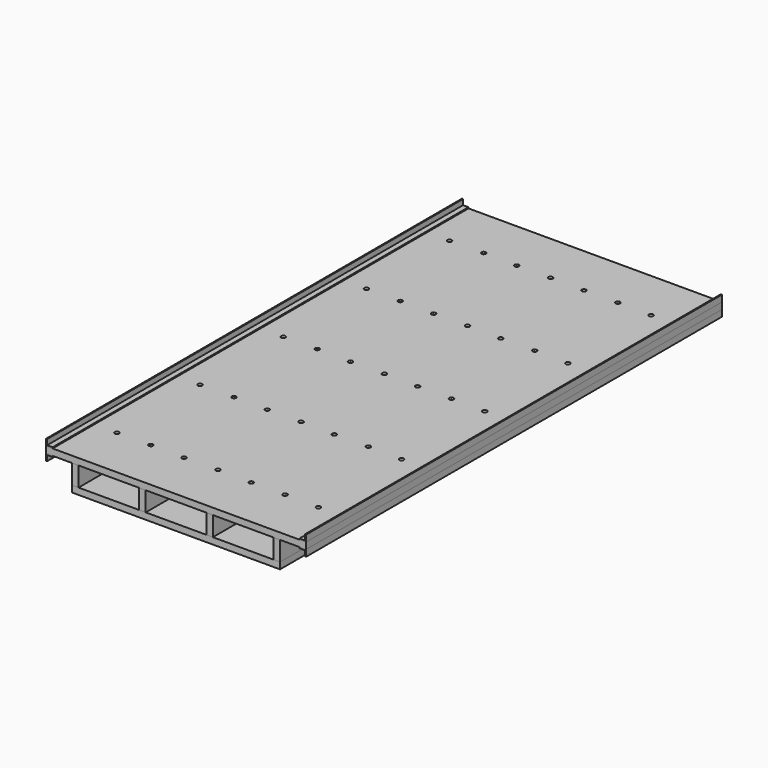
from build123d import *

# Parameters (mm, degrees)
F0_W                     = 762
F0_H                     = 1524
F1_DEPTH                 = 19.05
F3_START                 = -19.05
F2_W                     = 19.05
F2_H                     = 1524
F3_DEPTH                 = 57.15
F5_START                 = -19.05
F4_W                     = 571.5
F4_H                     = 19.05
F5_DEPTH                 = 57.15
F6_W                     = 19.05
F6_H                     = 28.575
F7_DEPTH                 = 1379.856
F11_D                    = 4.7625
F11_DEPTH                = 38.1
F11_CSINK_D              = 12.7
F11_CSINK_ANGLE          = 90
F11_TIP                  = 1.4307993491
F11_2_D                  = 4.7625
F11_2_DEPTH              = 38.1
F11_2_CSINK_D            = 12.7
F11_2_CSINK_ANGLE        = 90
F11_2_TIP                = 1.4307993491
F11_3_D                  = 4.7625
F11_3_DEPTH              = 38.1
F11_3_CSINK_D            = 12.7
F11_3_CSINK_ANGLE        = 90
F11_3_TIP                = 1.4307993491
F11_4_D                  = 4.7625
F11_4_DEPTH              = 38.1
F11_4_CSINK_D            = 12.7
F11_4_CSINK_ANGLE        = 90
F11_4_TIP                = 1.4307993491
F11_5_D                  = 4.7625
F11_5_DEPTH              = 38.1
F11_5_CSINK_D            = 12.7
F11_5_CSINK_ANGLE        = 90
F11_5_TIP                = 1.4307993491
F11_ON_F10_D             = 4.7625
F11_ON_F10_DEPTH         = 38.1
F11_ON_F10_CSINK_D       = 12.7
F11_ON_F10_CSINK_ANGLE   = 90
F11_ON_F10_TIP           = 1.4307993491
F12_W                    = 609.6
F12_H                    = 1524
F13_DEPTH                = 19.05
F15_D                    = 4.7625
F15_DEPTH                = 38.1
F15_CSINK_D              = 12.7
F15_CSINK_ANGLE          = 90
F15_TIP                  = 1.4307993491
F15_2_D                  = 4.7625
F15_2_DEPTH              = 38.1
F15_2_CSINK_D            = 12.7
F15_2_CSINK_ANGLE        = 90
F15_2_TIP                = 1.4307993491
F15_3_D                  = 4.7625
F15_3_DEPTH              = 38.1
F15_3_CSINK_D            = 12.7
F15_3_CSINK_ANGLE        = 90
F15_3_TIP                = 1.4307993491
F15_4_D                  = 4.7625
F15_4_DEPTH              = 38.1
F15_4_CSINK_D            = 12.7
F15_4_CSINK_ANGLE        = 90
F15_4_TIP                = 1.4307993491
F15_5_D                  = 4.7625
F15_5_DEPTH              = 38.1
F15_5_CSINK_D            = 12.7
F15_5_CSINK_ANGLE        = 90
F15_5_TIP                = 1.4307993491
F15_6_D                  = 4.7625
F15_6_DEPTH              = 38.1
F15_6_CSINK_D            = 12.7
F15_6_CSINK_ANGLE        = 90
F15_6_TIP                = 1.4307993491
F15_7_D                  = 4.7625
F15_7_DEPTH              = 38.1
F15_7_CSINK_D            = 12.7
F15_7_CSINK_ANGLE        = 90
F15_7_TIP                = 1.4307993491
F15_8_D                  = 4.7625
F15_8_DEPTH              = 38.1
F15_8_CSINK_D            = 12.7
F15_8_CSINK_ANGLE        = 90
F15_8_TIP                = 1.4307993491
F17_D                    = 4.7625
F17_DEPTH                = 38.1
F17_CSINK_D              = 12.7
F17_CSINK_ANGLE          = 90
F17_TIP                  = 1.4307993491
F17_2_D                  = 4.7625
F17_2_DEPTH              = 38.1
F17_2_CSINK_D            = 12.7
F17_2_CSINK_ANGLE        = 90
F17_2_TIP                = 1.4307993491
F17_3_D                  = 4.7625
F17_3_DEPTH              = 38.1
F17_3_CSINK_D            = 12.7
F17_3_CSINK_ANGLE        = 90
F17_3_TIP                = 1.4307993491
F17_4_D                  = 4.7625
F17_4_DEPTH              = 38.1
F17_4_CSINK_D            = 12.7
F17_4_CSINK_ANGLE        = 90
F17_4_TIP                = 1.4307993491
F17_5_D                  = 4.7625
F17_5_DEPTH              = 38.1
F17_5_CSINK_D            = 12.7
F17_5_CSINK_ANGLE        = 90
F17_5_TIP                = 1.4307993491
F17_6_D                  = 4.7625
F17_6_DEPTH              = 38.1
F17_6_CSINK_D            = 12.7
F17_6_CSINK_ANGLE        = 90
F17_6_TIP                = 1.4307993491
F19_D                    = 4.7625
F19_DEPTH                = 38.1
F19_START                = 19.05
F19_CSINK_D              = 12.7
F19_CSINK_ANGLE          = 90
F19_TIP                  = 1.4307993491
F19_2_D                  = 4.7625
F19_2_DEPTH              = 38.1
F19_2_START              = 19.05
F19_2_CSINK_D            = 12.7
F19_2_CSINK_ANGLE        = 90
F19_2_TIP                = 1.4307993491
F19_3_D                  = 4.7625
F19_3_DEPTH              = 38.1
F19_3_START              = 19.05
F19_3_CSINK_D            = 12.7
F19_3_CSINK_ANGLE        = 90
F19_3_TIP                = 1.4307993491
F19_4_D                  = 4.7625
F19_4_DEPTH              = 38.1
F19_4_START              = 19.05
F19_4_CSINK_D            = 12.7
F19_4_CSINK_ANGLE        = 90
F19_4_TIP                = 1.4307993491
F19_5_D                  = 4.7625
F19_5_DEPTH              = 38.1
F19_5_START              = 19.05
F19_5_CSINK_D            = 12.7
F19_5_CSINK_ANGLE        = 90
F19_5_TIP                = 1.4307993491
F19_ON_F18_D             = 4.7625
F19_ON_F18_DEPTH         = 38.1
F19_ON_F18_CSINK_D       = 12.7
F19_ON_F18_CSINK_ANGLE   = 90
F19_ON_F18_TIP           = 1.4307993491
F19_ON_F18_2_D           = 4.7625
F19_ON_F18_2_DEPTH       = 38.1
F19_ON_F18_2_CSINK_D     = 12.7
F19_ON_F18_2_CSINK_ANGLE = 90
F19_ON_F18_2_TIP         = 1.4307993491
F19_ON_F18_3_D           = 4.7625
F19_ON_F18_3_DEPTH       = 38.1
F19_ON_F18_3_CSINK_D     = 12.7
F19_ON_F18_3_CSINK_ANGLE = 90
F19_ON_F18_3_TIP         = 1.4307993491
F19_ON_F18_4_D           = 4.7625
F19_ON_F18_4_DEPTH       = 38.1
F19_ON_F18_4_CSINK_D     = 12.7
F19_ON_F18_4_CSINK_ANGLE = 90
F19_ON_F18_4_TIP         = 1.4307993491
F19_ON_F18_5_D           = 4.7625
F19_ON_F18_5_DEPTH       = 38.1
F19_ON_F18_5_CSINK_D     = 12.7
F19_ON_F18_5_CSINK_ANGLE = 90
F19_ON_F18_5_TIP         = 1.4307993491
F19_ON_F18_6_D           = 4.7625
F19_ON_F18_6_DEPTH       = 38.1
F19_ON_F18_6_CSINK_D     = 12.7
F19_ON_F18_6_CSINK_ANGLE = 90
F19_ON_F18_6_TIP         = 1.4307993491
F21_DEPTH                = 1524


# Not quite as in the source:
# - a feature names something its author has since deleted; it is built from what else it names


with BuildPart() as f1:
    # F0 (on Top) → F1 (new body)
    with BuildSketch(Plane.XY):
        with Locations((381, 762)):
            Rectangle(F0_W, F0_H)
    extrude(amount=-F1_DEPTH)

    # F11
    with Locations(Plane.XY):
        with Locations((85.725, 457.2), (85.725, 762), (85.725, 1066.8), (85.725, 1371.6), (676.275, 1066.8), (479.425, 1371.6), (479.425, 1066.8), (479.425, 762), (479.425, 457.2), (282.575, 1371.6), (479.425, 152.4), (676.275, 457.2), (282.575, 762), (676.275, 152.4), (282.575, 1066.8), (282.575, 152.4), (676.275, 762), (282.575, 457.2), (676.275, 1371.6), (85.725, 152.4)):
            CounterSinkHole(F11_D / 2, F11_CSINK_D / 2, depth=F11_DEPTH, counter_sink_angle=F11_CSINK_ANGLE)
            with Locations((0, 0, -(F11_DEPTH + F11_TIP / 2))):  # 118° drill point
                Cone(0, F11_D / 2, F11_TIP, mode=Mode.SUBTRACT)

    # F11 on F10
    with Locations(Plane.XY):
        with Locations((184.15, 1068.07), (381, 1372.87), (381, 153.67), (577.85, 1372.87), (381, 763.27), (184.15, 458.47), (184.15, 763.27), (577.85, 153.67), (577.85, 763.27), (381, 458.47), (184.15, 153.67), (577.85, 458.47), (184.15, 1372.87), (577.85, 1068.07), (381, 1068.07)):
            CounterSinkHole(F11_ON_F10_D / 2, F11_ON_F10_CSINK_D / 2, depth=F11_ON_F10_DEPTH, counter_sink_angle=F11_ON_F10_CSINK_ANGLE)
            with Locations((0, 0, -(F11_ON_F10_DEPTH + F11_ON_F10_TIP / 2))):  # 118° drill point
                Cone(0, F11_ON_F10_D / 2, F11_ON_F10_TIP, mode=Mode.SUBTRACT)


with BuildPart() as f3:
    # F2 (on face) → F3 (new body)
    with BuildSketch(Plane.XY.offset(F3_START)):
        with Locations((85.725, 762)):
            Rectangle(F2_W, F2_H)
    extrude(amount=-F3_DEPTH)

    # F11#2
    with Locations(Plane.XY):
        with Locations((85.725, 457.2), (85.725, 762), (85.725, 1066.8), (85.725, 1371.6), (676.275, 1066.8), (479.425, 1371.6), (479.425, 1066.8), (479.425, 762), (479.425, 457.2), (282.575, 1371.6), (479.425, 152.4), (676.275, 457.2), (282.575, 762), (676.275, 152.4), (282.575, 1066.8), (282.575, 152.4), (676.275, 762), (282.575, 457.2), (676.275, 1371.6), (85.725, 152.4)):
            CounterSinkHole(F11_2_D / 2, F11_2_CSINK_D / 2, depth=F11_2_DEPTH, counter_sink_angle=F11_2_CSINK_ANGLE)
            with Locations((0, 0, -(F11_2_DEPTH + F11_2_TIP / 2))):  # 118° drill point
                Cone(0, F11_2_D / 2, F11_2_TIP, mode=Mode.SUBTRACT)

    # F15
    with Locations(Plane(origin=(0, 0, -95.25), x_dir=(1, 0, 0), z_dir=(0, 0, -1))):
        with Locations((184.15, -152.4), (381, -458.47), (381, -763.27), (676.275, -762), (184.15, -458.47), (282.575, -762), (381, -153.67), (479.425, -762), (282.575, -457.2), (676.275, -457.2), (479.425, -457.2), (577.85, -153.67), (479.425, -152.4), (676.275, -152.4), (282.575, -153.67), (577.85, -458.47), (577.85, -763.27), (282.575, -1371.6), (676.275, -1066.8), (85.725, -1066.8), (479.425, -1371.6), (85.725, -152.4), (479.425, -1066.8), (577.85, -1372.87), (282.575, -1066.8), (381, -1068.07), (381, -1372.87), (85.725, -762), (577.85, -1068.07), (85.725, -457.2), (184.15, -1372.87), (85.725, -1371.6), (676.275, -1371.6), (184.15, -1068.07), (184.15, -762)):
            CounterSinkHole(F15_D / 2, F15_CSINK_D / 2, depth=F15_DEPTH, counter_sink_angle=F15_CSINK_ANGLE)
            with Locations((0, 0, -(F15_DEPTH + F15_TIP / 2))):  # 118° drill point
                Cone(0, F15_D / 2, F15_TIP, mode=Mode.SUBTRACT)

    # F17
    with Locations(Plane(origin=(76.2, 0, 0), x_dir=(0, -1, 0), z_dir=(-1, 0, 0))):
        with Locations((-458.47, -57.15), (-1372.87, -38.1), (-1372.87, -57.15), (-458.47, -38.1), (-1068.07, -57.15), (-763.27, -38.1), (-153.67, -57.15), (-1068.07, -38.1), (-763.27, -57.15), (-153.67, -38.1)):
            CounterSinkHole(F17_D / 2, F17_CSINK_D / 2, depth=F17_DEPTH, counter_sink_angle=F17_CSINK_ANGLE)
            with Locations((0, 0, -(F17_DEPTH + F17_TIP / 2))):  # 118° drill point
                Cone(0, F17_D / 2, F17_TIP, mode=Mode.SUBTRACT)


with BuildPart() as f3b:
    # F2 (on face) → F3, piece 2 (new body)
    with BuildSketch(Plane.XY.offset(F3_START)):
        with Locations((282.575, 762)):
            Rectangle(F2_W, F2_H)
    extrude(amount=-F3_DEPTH)


with BuildPart() as f3c:
    # F2 (on face) → F3, piece 3 (new body)
    with BuildSketch(Plane.XY.offset(F3_START)):
        with Locations((479.425, 762)):
            Rectangle(F2_W, F2_H)
    extrude(amount=-F3_DEPTH)


with BuildPart() as f3d:
    # F2 (on face) → F3, piece 4 (new body)
    with BuildSketch(Plane.XY.offset(F3_START)):
        with Locations((676.275, 762)):
            Rectangle(F2_W, F2_H)
    extrude(amount=-F3_DEPTH)

    # F11#5
    with Locations(Plane.XY):
        with Locations((85.725, 457.2), (85.725, 762), (85.725, 1066.8), (85.725, 1371.6), (676.275, 1066.8), (479.425, 1371.6), (479.425, 1066.8), (479.425, 762), (479.425, 457.2), (282.575, 1371.6), (479.425, 152.4), (676.275, 457.2), (282.575, 762), (676.275, 152.4), (282.575, 1066.8), (282.575, 152.4), (676.275, 762), (282.575, 457.2), (676.275, 1371.6), (85.725, 152.4)):
            CounterSinkHole(F11_5_D / 2, F11_5_CSINK_D / 2, depth=F11_5_DEPTH, counter_sink_angle=F11_5_CSINK_ANGLE)
            with Locations((0, 0, -(F11_5_DEPTH + F11_5_TIP / 2))):  # 118° drill point
                Cone(0, F11_5_D / 2, F11_5_TIP, mode=Mode.SUBTRACT)

    # F15#2
    with Locations(Plane(origin=(0, 0, -95.25), x_dir=(1, 0, 0), z_dir=(0, 0, -1))):
        with Locations((184.15, -152.4), (381, -458.47), (381, -763.27), (676.275, -762), (184.15, -458.47), (282.575, -762), (381, -153.67), (479.425, -762), (282.575, -457.2), (676.275, -457.2), (479.425, -457.2), (577.85, -153.67), (479.425, -152.4), (676.275, -152.4), (282.575, -153.67), (577.85, -458.47), (577.85, -763.27), (282.575, -1371.6), (676.275, -1066.8), (85.725, -1066.8), (479.425, -1371.6), (85.725, -152.4), (479.425, -1066.8), (577.85, -1372.87), (282.575, -1066.8), (381, -1068.07), (381, -1372.87), (85.725, -762), (577.85, -1068.07), (85.725, -457.2), (184.15, -1372.87), (85.725, -1371.6), (676.275, -1371.6), (184.15, -1068.07), (184.15, -762)):
            CounterSinkHole(F15_2_D / 2, F15_2_CSINK_D / 2, depth=F15_2_DEPTH, counter_sink_angle=F15_2_CSINK_ANGLE)
            with Locations((0, 0, -(F15_2_DEPTH + F15_2_TIP / 2))):  # 118° drill point
                Cone(0, F15_2_D / 2, F15_2_TIP, mode=Mode.SUBTRACT)

    # F19 on F18
    with Locations(Plane.YZ.offset(685.8)):
        with Locations((763.27, -38.1), (458.47, -38.1), (153.67, -57.15), (1068.07, -57.15), (153.67, -38.1), (458.47, -57.15), (1372.87, -38.1), (1372.87, -57.15), (1068.07, -38.1), (763.27, -57.15)):
            CounterSinkHole(F19_ON_F18_D / 2, F19_ON_F18_CSINK_D / 2, depth=F19_ON_F18_DEPTH, counter_sink_angle=F19_ON_F18_CSINK_ANGLE)
            with Locations((0, 0, -(F19_ON_F18_DEPTH + F19_ON_F18_TIP / 2))):  # 118° drill point
                Cone(0, F19_ON_F18_D / 2, F19_ON_F18_TIP, mode=Mode.SUBTRACT)


with BuildPart() as f5:
    # F4 (on face) → F5 (new body)
    with BuildSketch(Plane.XY.offset(F5_START)):
        with Locations((381, 153.67)):
            Rectangle(F4_W, F4_H)
    extrude(amount=-F5_DEPTH)


with BuildPart() as f5b:
    # F4 (on face) → F5, piece 2 (new body)
    with BuildSketch(Plane.XY.offset(F5_START)):
        with Locations((381, 763.27)):
            Rectangle(F4_W, F4_H)
    extrude(amount=-F5_DEPTH)


with BuildPart() as f5c:
    # F4 (on face) → F5, piece 3 (new body)
    with BuildSketch(Plane.XY.offset(F5_START)):
        with Locations((381, 1068.07)):
            Rectangle(F4_W, F4_H)
    extrude(amount=-F5_DEPTH)


with BuildPart() as f5d:
    # F4 (on face) → F5, piece 4 (new body)
    with BuildSketch(Plane.XY.offset(F5_START)):
        with Locations((381, 1372.87)):
            Rectangle(F4_W, F4_H)
    extrude(amount=-F5_DEPTH)


with BuildPart() as f5e:
    # F4 (on face) → F5, piece 5 (new body)
    with BuildSketch(Plane.XY.offset(F5_START)):
        with Locations((381, 458.47)):
            Rectangle(F4_W, F4_H)
    extrude(amount=-F5_DEPTH)


with BuildPart() as f7_tool:
    # F6 (on face) → F7 (new body, through all)
    with BuildSketch(Plane.XZ.offset(-144.145)):
        with Locations((282.575, -33.3375)):
            Rectangle(F6_W, F6_H)
        with Locations((479.425, -33.3375)):
            Rectangle(F6_W, F6_H)
    extrude(amount=-F7_DEPTH)


with BuildPart() as f5_1:
    add(f5.part)

    # F7: cut by f7_tool
    add(f7_tool.part, mode=Mode.SUBTRACT)


with BuildPart() as f5b_1:
    add(f5b.part)

    # F7: cut by f7_tool
    add(f7_tool.part, mode=Mode.SUBTRACT)


with BuildPart() as f5c_1:
    add(f5c.part)

    # F7: cut by f7_tool
    add(f7_tool.part, mode=Mode.SUBTRACT)


with BuildPart() as f5d_1:
    add(f5d.part)

    # F7: cut by f7_tool
    add(f7_tool.part, mode=Mode.SUBTRACT)


with BuildPart() as f5e_1:
    add(f5e.part)

    # F7: cut by f7_tool
    add(f7_tool.part, mode=Mode.SUBTRACT)


with BuildPart() as f3b_1:
    add(f3b.part)

    # F8: cut F5, F5e, F5b, F5c, F5d
    add(f5_1.part, mode=Mode.SUBTRACT)
    add(f5e_1.part, mode=Mode.SUBTRACT)
    add(f5b_1.part, mode=Mode.SUBTRACT)
    add(f5c_1.part, mode=Mode.SUBTRACT)
    add(f5d_1.part, mode=Mode.SUBTRACT)

    # F11#3
    with Locations(Plane.XY):
        with Locations((85.725, 457.2), (85.725, 762), (85.725, 1066.8), (85.725, 1371.6), (676.275, 1066.8), (479.425, 1371.6), (479.425, 1066.8), (479.425, 762), (479.425, 457.2), (282.575, 1371.6), (479.425, 152.4), (676.275, 457.2), (282.575, 762), (676.275, 152.4), (282.575, 1066.8), (282.575, 152.4), (676.275, 762), (282.575, 457.2), (676.275, 1371.6), (85.725, 152.4)):
            CounterSinkHole(F11_3_D / 2, F11_3_CSINK_D / 2, depth=F11_3_DEPTH, counter_sink_angle=F11_3_CSINK_ANGLE)
            with Locations((0, 0, -(F11_3_DEPTH + F11_3_TIP / 2))):  # 118° drill point
                Cone(0, F11_3_D / 2, F11_3_TIP, mode=Mode.SUBTRACT)


with BuildPart() as f3c_1:
    add(f3c.part)

    # F8: cut F5, F5e, F5b, F5c, F5d
    add(f5_1.part, mode=Mode.SUBTRACT)
    add(f5e_1.part, mode=Mode.SUBTRACT)
    add(f5b_1.part, mode=Mode.SUBTRACT)
    add(f5c_1.part, mode=Mode.SUBTRACT)
    add(f5d_1.part, mode=Mode.SUBTRACT)

    # F11#4
    with Locations(Plane.XY):
        with Locations((85.725, 457.2), (85.725, 762), (85.725, 1066.8), (85.725, 1371.6), (676.275, 1066.8), (479.425, 1371.6), (479.425, 1066.8), (479.425, 762), (479.425, 457.2), (282.575, 1371.6), (479.425, 152.4), (676.275, 457.2), (282.575, 762), (676.275, 152.4), (282.575, 1066.8), (282.575, 152.4), (676.275, 762), (282.575, 457.2), (676.275, 1371.6), (85.725, 152.4)):
            CounterSinkHole(F11_4_D / 2, F11_4_CSINK_D / 2, depth=F11_4_DEPTH, counter_sink_angle=F11_4_CSINK_ANGLE)
            with Locations((0, 0, -(F11_4_DEPTH + F11_4_TIP / 2))):  # 118° drill point
                Cone(0, F11_4_D / 2, F11_4_TIP, mode=Mode.SUBTRACT)


with BuildPart() as f13:
    # F12 (on face) → F13 (new body)
    with BuildSketch(Plane(origin=(0, 0, -76.2), x_dir=(1, 0, 0), z_dir=(0, 0, -1))):
        with Locations((381, -762)):
            Rectangle(F12_W, F12_H)
    extrude(amount=F13_DEPTH)

    # F15#8
    with Locations(Plane(origin=(0, 0, -95.25), x_dir=(1, 0, 0), z_dir=(0, 0, -1))):
        with Locations((184.15, -152.4), (381, -458.47), (381, -763.27), (676.275, -762), (184.15, -458.47), (282.575, -762), (381, -153.67), (479.425, -762), (282.575, -457.2), (676.275, -457.2), (479.425, -457.2), (577.85, -153.67), (479.425, -152.4), (676.275, -152.4), (282.575, -153.67), (577.85, -458.47), (577.85, -763.27), (282.575, -1371.6), (676.275, -1066.8), (85.725, -1066.8), (479.425, -1371.6), (85.725, -152.4), (479.425, -1066.8), (577.85, -1372.87), (282.575, -1066.8), (381, -1068.07), (381, -1372.87), (85.725, -762), (577.85, -1068.07), (85.725, -457.2), (184.15, -1372.87), (85.725, -1371.6), (676.275, -1371.6), (184.15, -1068.07), (184.15, -762)):
            CounterSinkHole(F15_8_D / 2, F15_8_CSINK_D / 2, depth=F15_8_DEPTH, counter_sink_angle=F15_8_CSINK_ANGLE)
            with Locations((0, 0, -(F15_8_DEPTH + F15_8_TIP / 2))):  # 118° drill point
                Cone(0, F15_8_D / 2, F15_8_TIP, mode=Mode.SUBTRACT)


with BuildPart() as f5_2:
    add(f5_1.part)

    # F15#3
    with Locations(Plane(origin=(0, 0, -95.25), x_dir=(1, 0, 0), z_dir=(0, 0, -1))):
        with Locations((184.15, -152.4), (381, -458.47), (381, -763.27), (676.275, -762), (184.15, -458.47), (282.575, -762), (381, -153.67), (479.425, -762), (282.575, -457.2), (676.275, -457.2), (479.425, -457.2), (577.85, -153.67), (479.425, -152.4), (676.275, -152.4), (282.575, -153.67), (577.85, -458.47), (577.85, -763.27), (282.575, -1371.6), (676.275, -1066.8), (85.725, -1066.8), (479.425, -1371.6), (85.725, -152.4), (479.425, -1066.8), (577.85, -1372.87), (282.575, -1066.8), (381, -1068.07), (381, -1372.87), (85.725, -762), (577.85, -1068.07), (85.725, -457.2), (184.15, -1372.87), (85.725, -1371.6), (676.275, -1371.6), (184.15, -1068.07), (184.15, -762)):
            CounterSinkHole(F15_3_D / 2, F15_3_CSINK_D / 2, depth=F15_3_DEPTH, counter_sink_angle=F15_3_CSINK_ANGLE)
            with Locations((0, 0, -(F15_3_DEPTH + F15_3_TIP / 2))):  # 118° drill point
                Cone(0, F15_3_D / 2, F15_3_TIP, mode=Mode.SUBTRACT)

    # F17#2
    with Locations(Plane(origin=(76.2, 0, 0), x_dir=(0, -1, 0), z_dir=(-1, 0, 0))):
        with Locations((-458.47, -57.15), (-1372.87, -38.1), (-1372.87, -57.15), (-458.47, -38.1), (-1068.07, -57.15), (-763.27, -38.1), (-153.67, -57.15), (-1068.07, -38.1), (-763.27, -57.15), (-153.67, -38.1)):
            CounterSinkHole(F17_2_D / 2, F17_2_CSINK_D / 2, depth=F17_2_DEPTH, counter_sink_angle=F17_2_CSINK_ANGLE)
            with Locations((0, 0, -(F17_2_DEPTH + F17_2_TIP / 2))):  # 118° drill point
                Cone(0, F17_2_D / 2, F17_2_TIP, mode=Mode.SUBTRACT)

    # F19
    # its depths count from where the whole tool has entered the part; down to there all is cleared
    with Locations(Plane(origin=(76.2, 0, 0), x_dir=(0, -1, 0), z_dir=(-1, 0, 0)).offset(-F19_START)):
        with Locations((-458.47, -57.15), (-1372.87, -38.1), (-1372.87, -57.15), (-458.47, -38.1), (-1068.07, -57.15), (-763.27, -38.1), (-153.67, -57.15), (-1068.07, -38.1), (-763.27, -57.15), (-153.67, -38.1)):
            CounterSinkHole(F19_D / 2, F19_CSINK_D / 2, depth=F19_DEPTH, counter_sink_angle=F19_CSINK_ANGLE)
            with Locations((0, 0, -(F19_DEPTH + F19_TIP / 2))):  # 118° drill point
                Cone(0, F19_D / 2, F19_TIP, mode=Mode.SUBTRACT)

    # F19 on F18#2
    with Locations(Plane.YZ.offset(685.8)):
        with Locations((763.27, -38.1), (458.47, -38.1), (153.67, -57.15), (1068.07, -57.15), (153.67, -38.1), (458.47, -57.15), (1372.87, -38.1), (1372.87, -57.15), (1068.07, -38.1), (763.27, -57.15)):
            CounterSinkHole(F19_ON_F18_2_D / 2, F19_ON_F18_2_CSINK_D / 2, depth=F19_ON_F18_2_DEPTH, counter_sink_angle=F19_ON_F18_2_CSINK_ANGLE)
            with Locations((0, 0, -(F19_ON_F18_2_DEPTH + F19_ON_F18_2_TIP / 2))):  # 118° drill point
                Cone(0, F19_ON_F18_2_D / 2, F19_ON_F18_2_TIP, mode=Mode.SUBTRACT)


with BuildPart() as f5b_2:
    add(f5b_1.part)

    # F15#4
    with Locations(Plane(origin=(0, 0, -95.25), x_dir=(1, 0, 0), z_dir=(0, 0, -1))):
        with Locations((184.15, -152.4), (381, -458.47), (381, -763.27), (676.275, -762), (184.15, -458.47), (282.575, -762), (381, -153.67), (479.425, -762), (282.575, -457.2), (676.275, -457.2), (479.425, -457.2), (577.85, -153.67), (479.425, -152.4), (676.275, -152.4), (282.575, -153.67), (577.85, -458.47), (577.85, -763.27), (282.575, -1371.6), (676.275, -1066.8), (85.725, -1066.8), (479.425, -1371.6), (85.725, -152.4), (479.425, -1066.8), (577.85, -1372.87), (282.575, -1066.8), (381, -1068.07), (381, -1372.87), (85.725, -762), (577.85, -1068.07), (85.725, -457.2), (184.15, -1372.87), (85.725, -1371.6), (676.275, -1371.6), (184.15, -1068.07), (184.15, -762)):
            CounterSinkHole(F15_4_D / 2, F15_4_CSINK_D / 2, depth=F15_4_DEPTH, counter_sink_angle=F15_4_CSINK_ANGLE)
            with Locations((0, 0, -(F15_4_DEPTH + F15_4_TIP / 2))):  # 118° drill point
                Cone(0, F15_4_D / 2, F15_4_TIP, mode=Mode.SUBTRACT)

    # F17#3
    with Locations(Plane(origin=(76.2, 0, 0), x_dir=(0, -1, 0), z_dir=(-1, 0, 0))):
        with Locations((-458.47, -57.15), (-1372.87, -38.1), (-1372.87, -57.15), (-458.47, -38.1), (-1068.07, -57.15), (-763.27, -38.1), (-153.67, -57.15), (-1068.07, -38.1), (-763.27, -57.15), (-153.67, -38.1)):
            CounterSinkHole(F17_3_D / 2, F17_3_CSINK_D / 2, depth=F17_3_DEPTH, counter_sink_angle=F17_3_CSINK_ANGLE)
            with Locations((0, 0, -(F17_3_DEPTH + F17_3_TIP / 2))):  # 118° drill point
                Cone(0, F17_3_D / 2, F17_3_TIP, mode=Mode.SUBTRACT)

    # F19#2
    # its depths count from where the whole tool has entered the part; down to there all is cleared
    with Locations(Plane(origin=(76.2, 0, 0), x_dir=(0, -1, 0), z_dir=(-1, 0, 0)).offset(-F19_2_START)):
        with Locations((-458.47, -57.15), (-1372.87, -38.1), (-1372.87, -57.15), (-458.47, -38.1), (-1068.07, -57.15), (-763.27, -38.1), (-153.67, -57.15), (-1068.07, -38.1), (-763.27, -57.15), (-153.67, -38.1)):
            CounterSinkHole(F19_2_D / 2, F19_2_CSINK_D / 2, depth=F19_2_DEPTH, counter_sink_angle=F19_2_CSINK_ANGLE)
            with Locations((0, 0, -(F19_2_DEPTH + F19_2_TIP / 2))):  # 118° drill point
                Cone(0, F19_2_D / 2, F19_2_TIP, mode=Mode.SUBTRACT)

    # F19 on F18#3
    with Locations(Plane.YZ.offset(685.8)):
        with Locations((763.27, -38.1), (458.47, -38.1), (153.67, -57.15), (1068.07, -57.15), (153.67, -38.1), (458.47, -57.15), (1372.87, -38.1), (1372.87, -57.15), (1068.07, -38.1), (763.27, -57.15)):
            CounterSinkHole(F19_ON_F18_3_D / 2, F19_ON_F18_3_CSINK_D / 2, depth=F19_ON_F18_3_DEPTH, counter_sink_angle=F19_ON_F18_3_CSINK_ANGLE)
            with Locations((0, 0, -(F19_ON_F18_3_DEPTH + F19_ON_F18_3_TIP / 2))):  # 118° drill point
                Cone(0, F19_ON_F18_3_D / 2, F19_ON_F18_3_TIP, mode=Mode.SUBTRACT)


with BuildPart() as f5c_2:
    add(f5c_1.part)

    # F15#5
    with Locations(Plane(origin=(0, 0, -95.25), x_dir=(1, 0, 0), z_dir=(0, 0, -1))):
        with Locations((184.15, -152.4), (381, -458.47), (381, -763.27), (676.275, -762), (184.15, -458.47), (282.575, -762), (381, -153.67), (479.425, -762), (282.575, -457.2), (676.275, -457.2), (479.425, -457.2), (577.85, -153.67), (479.425, -152.4), (676.275, -152.4), (282.575, -153.67), (577.85, -458.47), (577.85, -763.27), (282.575, -1371.6), (676.275, -1066.8), (85.725, -1066.8), (479.425, -1371.6), (85.725, -152.4), (479.425, -1066.8), (577.85, -1372.87), (282.575, -1066.8), (381, -1068.07), (381, -1372.87), (85.725, -762), (577.85, -1068.07), (85.725, -457.2), (184.15, -1372.87), (85.725, -1371.6), (676.275, -1371.6), (184.15, -1068.07), (184.15, -762)):
            CounterSinkHole(F15_5_D / 2, F15_5_CSINK_D / 2, depth=F15_5_DEPTH, counter_sink_angle=F15_5_CSINK_ANGLE)
            with Locations((0, 0, -(F15_5_DEPTH + F15_5_TIP / 2))):  # 118° drill point
                Cone(0, F15_5_D / 2, F15_5_TIP, mode=Mode.SUBTRACT)

    # F17#4
    with Locations(Plane(origin=(76.2, 0, 0), x_dir=(0, -1, 0), z_dir=(-1, 0, 0))):
        with Locations((-458.47, -57.15), (-1372.87, -38.1), (-1372.87, -57.15), (-458.47, -38.1), (-1068.07, -57.15), (-763.27, -38.1), (-153.67, -57.15), (-1068.07, -38.1), (-763.27, -57.15), (-153.67, -38.1)):
            CounterSinkHole(F17_4_D / 2, F17_4_CSINK_D / 2, depth=F17_4_DEPTH, counter_sink_angle=F17_4_CSINK_ANGLE)
            with Locations((0, 0, -(F17_4_DEPTH + F17_4_TIP / 2))):  # 118° drill point
                Cone(0, F17_4_D / 2, F17_4_TIP, mode=Mode.SUBTRACT)

    # F19#3
    # its depths count from where the whole tool has entered the part; down to there all is cleared
    with Locations(Plane(origin=(76.2, 0, 0), x_dir=(0, -1, 0), z_dir=(-1, 0, 0)).offset(-F19_3_START)):
        with Locations((-458.47, -57.15), (-1372.87, -38.1), (-1372.87, -57.15), (-458.47, -38.1), (-1068.07, -57.15), (-763.27, -38.1), (-153.67, -57.15), (-1068.07, -38.1), (-763.27, -57.15), (-153.67, -38.1)):
            CounterSinkHole(F19_3_D / 2, F19_3_CSINK_D / 2, depth=F19_3_DEPTH, counter_sink_angle=F19_3_CSINK_ANGLE)
            with Locations((0, 0, -(F19_3_DEPTH + F19_3_TIP / 2))):  # 118° drill point
                Cone(0, F19_3_D / 2, F19_3_TIP, mode=Mode.SUBTRACT)

    # F19 on F18#4
    with Locations(Plane.YZ.offset(685.8)):
        with Locations((763.27, -38.1), (458.47, -38.1), (153.67, -57.15), (1068.07, -57.15), (153.67, -38.1), (458.47, -57.15), (1372.87, -38.1), (1372.87, -57.15), (1068.07, -38.1), (763.27, -57.15)):
            CounterSinkHole(F19_ON_F18_4_D / 2, F19_ON_F18_4_CSINK_D / 2, depth=F19_ON_F18_4_DEPTH, counter_sink_angle=F19_ON_F18_4_CSINK_ANGLE)
            with Locations((0, 0, -(F19_ON_F18_4_DEPTH + F19_ON_F18_4_TIP / 2))):  # 118° drill point
                Cone(0, F19_ON_F18_4_D / 2, F19_ON_F18_4_TIP, mode=Mode.SUBTRACT)


with BuildPart() as f5d_2:
    add(f5d_1.part)

    # F15#6
    with Locations(Plane(origin=(0, 0, -95.25), x_dir=(1, 0, 0), z_dir=(0, 0, -1))):
        with Locations((184.15, -152.4), (381, -458.47), (381, -763.27), (676.275, -762), (184.15, -458.47), (282.575, -762), (381, -153.67), (479.425, -762), (282.575, -457.2), (676.275, -457.2), (479.425, -457.2), (577.85, -153.67), (479.425, -152.4), (676.275, -152.4), (282.575, -153.67), (577.85, -458.47), (577.85, -763.27), (282.575, -1371.6), (676.275, -1066.8), (85.725, -1066.8), (479.425, -1371.6), (85.725, -152.4), (479.425, -1066.8), (577.85, -1372.87), (282.575, -1066.8), (381, -1068.07), (381, -1372.87), (85.725, -762), (577.85, -1068.07), (85.725, -457.2), (184.15, -1372.87), (85.725, -1371.6), (676.275, -1371.6), (184.15, -1068.07), (184.15, -762)):
            CounterSinkHole(F15_6_D / 2, F15_6_CSINK_D / 2, depth=F15_6_DEPTH, counter_sink_angle=F15_6_CSINK_ANGLE)
            with Locations((0, 0, -(F15_6_DEPTH + F15_6_TIP / 2))):  # 118° drill point
                Cone(0, F15_6_D / 2, F15_6_TIP, mode=Mode.SUBTRACT)

    # F17#5
    with Locations(Plane(origin=(76.2, 0, 0), x_dir=(0, -1, 0), z_dir=(-1, 0, 0))):
        with Locations((-458.47, -57.15), (-1372.87, -38.1), (-1372.87, -57.15), (-458.47, -38.1), (-1068.07, -57.15), (-763.27, -38.1), (-153.67, -57.15), (-1068.07, -38.1), (-763.27, -57.15), (-153.67, -38.1)):
            CounterSinkHole(F17_5_D / 2, F17_5_CSINK_D / 2, depth=F17_5_DEPTH, counter_sink_angle=F17_5_CSINK_ANGLE)
            with Locations((0, 0, -(F17_5_DEPTH + F17_5_TIP / 2))):  # 118° drill point
                Cone(0, F17_5_D / 2, F17_5_TIP, mode=Mode.SUBTRACT)

    # F19#4
    # its depths count from where the whole tool has entered the part; down to there all is cleared
    with Locations(Plane(origin=(76.2, 0, 0), x_dir=(0, -1, 0), z_dir=(-1, 0, 0)).offset(-F19_4_START)):
        with Locations((-458.47, -57.15), (-1372.87, -38.1), (-1372.87, -57.15), (-458.47, -38.1), (-1068.07, -57.15), (-763.27, -38.1), (-153.67, -57.15), (-1068.07, -38.1), (-763.27, -57.15), (-153.67, -38.1)):
            CounterSinkHole(F19_4_D / 2, F19_4_CSINK_D / 2, depth=F19_4_DEPTH, counter_sink_angle=F19_4_CSINK_ANGLE)
            with Locations((0, 0, -(F19_4_DEPTH + F19_4_TIP / 2))):  # 118° drill point
                Cone(0, F19_4_D / 2, F19_4_TIP, mode=Mode.SUBTRACT)

    # F19 on F18#5
    with Locations(Plane.YZ.offset(685.8)):
        with Locations((763.27, -38.1), (458.47, -38.1), (153.67, -57.15), (1068.07, -57.15), (153.67, -38.1), (458.47, -57.15), (1372.87, -38.1), (1372.87, -57.15), (1068.07, -38.1), (763.27, -57.15)):
            CounterSinkHole(F19_ON_F18_5_D / 2, F19_ON_F18_5_CSINK_D / 2, depth=F19_ON_F18_5_DEPTH, counter_sink_angle=F19_ON_F18_5_CSINK_ANGLE)
            with Locations((0, 0, -(F19_ON_F18_5_DEPTH + F19_ON_F18_5_TIP / 2))):  # 118° drill point
                Cone(0, F19_ON_F18_5_D / 2, F19_ON_F18_5_TIP, mode=Mode.SUBTRACT)


with BuildPart() as f5e_2:
    add(f5e_1.part)

    # F15#7
    with Locations(Plane(origin=(0, 0, -95.25), x_dir=(1, 0, 0), z_dir=(0, 0, -1))):
        with Locations((184.15, -152.4), (381, -458.47), (381, -763.27), (676.275, -762), (184.15, -458.47), (282.575, -762), (381, -153.67), (479.425, -762), (282.575, -457.2), (676.275, -457.2), (479.425, -457.2), (577.85, -153.67), (479.425, -152.4), (676.275, -152.4), (282.575, -153.67), (577.85, -458.47), (577.85, -763.27), (282.575, -1371.6), (676.275, -1066.8), (85.725, -1066.8), (479.425, -1371.6), (85.725, -152.4), (479.425, -1066.8), (577.85, -1372.87), (282.575, -1066.8), (381, -1068.07), (381, -1372.87), (85.725, -762), (577.85, -1068.07), (85.725, -457.2), (184.15, -1372.87), (85.725, -1371.6), (676.275, -1371.6), (184.15, -1068.07), (184.15, -762)):
            CounterSinkHole(F15_7_D / 2, F15_7_CSINK_D / 2, depth=F15_7_DEPTH, counter_sink_angle=F15_7_CSINK_ANGLE)
            with Locations((0, 0, -(F15_7_DEPTH + F15_7_TIP / 2))):  # 118° drill point
                Cone(0, F15_7_D / 2, F15_7_TIP, mode=Mode.SUBTRACT)

    # F17#6
    with Locations(Plane(origin=(76.2, 0, 0), x_dir=(0, -1, 0), z_dir=(-1, 0, 0))):
        with Locations((-458.47, -57.15), (-1372.87, -38.1), (-1372.87, -57.15), (-458.47, -38.1), (-1068.07, -57.15), (-763.27, -38.1), (-153.67, -57.15), (-1068.07, -38.1), (-763.27, -57.15), (-153.67, -38.1)):
            CounterSinkHole(F17_6_D / 2, F17_6_CSINK_D / 2, depth=F17_6_DEPTH, counter_sink_angle=F17_6_CSINK_ANGLE)
            with Locations((0, 0, -(F17_6_DEPTH + F17_6_TIP / 2))):  # 118° drill point
                Cone(0, F17_6_D / 2, F17_6_TIP, mode=Mode.SUBTRACT)

    # F19#5
    # its depths count from where the whole tool has entered the part; down to there all is cleared
    with Locations(Plane(origin=(76.2, 0, 0), x_dir=(0, -1, 0), z_dir=(-1, 0, 0)).offset(-F19_5_START)):
        with Locations((-458.47, -57.15), (-1372.87, -38.1), (-1372.87, -57.15), (-458.47, -38.1), (-1068.07, -57.15), (-763.27, -38.1), (-153.67, -57.15), (-1068.07, -38.1), (-763.27, -57.15), (-153.67, -38.1)):
            CounterSinkHole(F19_5_D / 2, F19_5_CSINK_D / 2, depth=F19_5_DEPTH, counter_sink_angle=F19_5_CSINK_ANGLE)
            with Locations((0, 0, -(F19_5_DEPTH + F19_5_TIP / 2))):  # 118° drill point
                Cone(0, F19_5_D / 2, F19_5_TIP, mode=Mode.SUBTRACT)

    # F19 on F18#6
    with Locations(Plane.YZ.offset(685.8)):
        with Locations((763.27, -38.1), (458.47, -38.1), (153.67, -57.15), (1068.07, -57.15), (153.67, -38.1), (458.47, -57.15), (1372.87, -38.1), (1372.87, -57.15), (1068.07, -38.1), (763.27, -57.15)):
            CounterSinkHole(F19_ON_F18_6_D / 2, F19_ON_F18_6_CSINK_D / 2, depth=F19_ON_F18_6_DEPTH, counter_sink_angle=F19_ON_F18_6_CSINK_ANGLE)
            with Locations((0, 0, -(F19_ON_F18_6_DEPTH + F19_ON_F18_6_TIP / 2))):  # 118° drill point
                Cone(0, F19_ON_F18_6_D / 2, F19_ON_F18_6_TIP, mode=Mode.SUBTRACT)


with BuildPart() as f21:
    # F20 (on face) → F21 (new body, through all)
    with BuildSketch(Plane.XZ):
        Polygon((742.95, 3.175), (742.95, 0), (762, 0), (762, 19.05), (758.825, 19.05), (758.825, 3.175), align=None)
    extrude(amount=-F21_DEPTH)


with BuildPart() as f21b:
    # F20 (on face) → F21, piece 2 (new body, through all)
    with BuildSketch(Plane.XZ):
        Polygon((762, -38.1), (762, -19.05), (742.95, -19.05), (742.95, -22.225), (758.825, -22.225), (758.825, -38.1), align=None)
    extrude(amount=-F21_DEPTH)


with BuildPart() as f21c:
    # F20 (on face) → F21, piece 3 (new body, through all)
    with BuildSketch(Plane.XZ):
        Polygon((19.05, -19.05), (0, -19.05), (0, -38.1), (3.175, -38.1), (3.175, -22.225), (19.05, -22.225), align=None)
    extrude(amount=-F21_DEPTH)


with BuildPart() as f21d:
    # F20 (on face) → F21, piece 4 (new body, through all)
    with BuildSketch(Plane.XZ):
        Polygon((0, 0), (19.05, 0), (19.05, 3.175), (3.175, 3.175), (3.175, 19.05), (0, 19.05), align=None)
    extrude(amount=-F21_DEPTH)


solid = Compound([f1.part, f3.part, f3d.part, f3b_1.part, f3c_1.part, f13.part, f5_2.part, f5b_2.part, f5c_2.part, f5d_2.part, f5e_2.part, f21.part, f21b.part, f21c.part, f21d.part])
